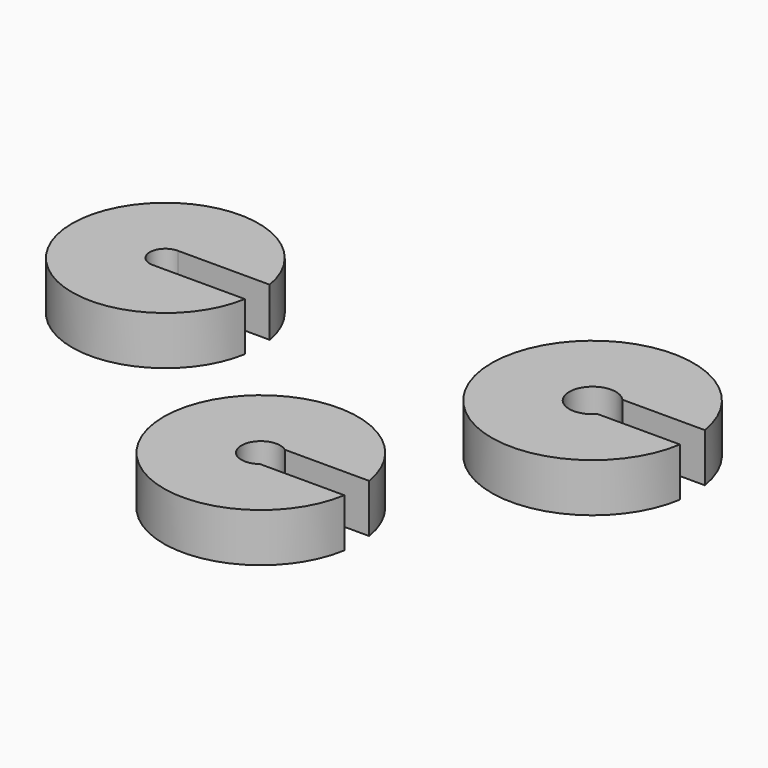
from build123d import *

# Parameters (mm, degrees)
F1_DEPTH = 3.175
F3_DEPTH = 3.175
F5_DEPTH = 3.175


# Not quite as in the source:
# - a length typed as a fraction of an inch, garbled in the dataset ("3 / 203.2 mm" for 3/8 in), is restored


with BuildPart() as f1:
    # F0 (on Top) → F1 (new body)
    with BuildSketch(Plane.XY):
        with BuildLine():
            ThreePointArc((0.762, -1.016), (-1.27, 0), (0.762, 1.016))
            Line((0.762, 1.016), (6.2681930411, 1.016))
            ThreePointArc((6.2681930411, 1.016), (-6.35, 0), (6.2681930411, -1.016))
            Line((6.2681930411, -1.016), (0.762, -1.016))
        make_face()
    extrude(amount=-F1_DEPTH)


with BuildPart() as f3:
    # F2 (on Top) → F3 (new body)
    with BuildSketch(Plane.XY):
        with BuildLine():
            ThreePointArc((14.5629012912, 9.3048050132), (11.9029787586, 10.3208050132), (14.5629012912, 11.3368050132))
            Line((14.5629012912, 11.3368050132), (19.9523569086, 11.3368050132))
            ThreePointArc((19.9523569086, 11.3368050132), (6.8229787586, 10.3208050132), (19.9523569086, 9.3048050132))
            Line((19.9523569086, 9.3048050132), (14.5629012912, 9.3048050132))
        make_face()
    extrude(amount=F3_DEPTH)


with BuildPart() as f5:
    # F4 (on Top) → F5 (new body)
    with BuildSketch(Plane.XY):
        with BuildLine():
            ThreePointArc((-13.4432689647, 7.9851497959), (-14.4592689667, 9.0011497959), (-13.4432689647, 10.0171497959))
            Line((-13.4432689647, 10.0171497959), (-7.4325319071, 10.0171497959))
            ThreePointArc((-7.4325319071, 10.0171497959), (-19.5392689667, 9.0011497959), (-7.4325319071, 7.9851497959))
            Line((-7.4325319071, 7.9851497959), (-13.4432689647, 7.9851497959))
        make_face()
    extrude(amount=F5_DEPTH)


solid = Compound([f1.part, f3.part, f5.part])
